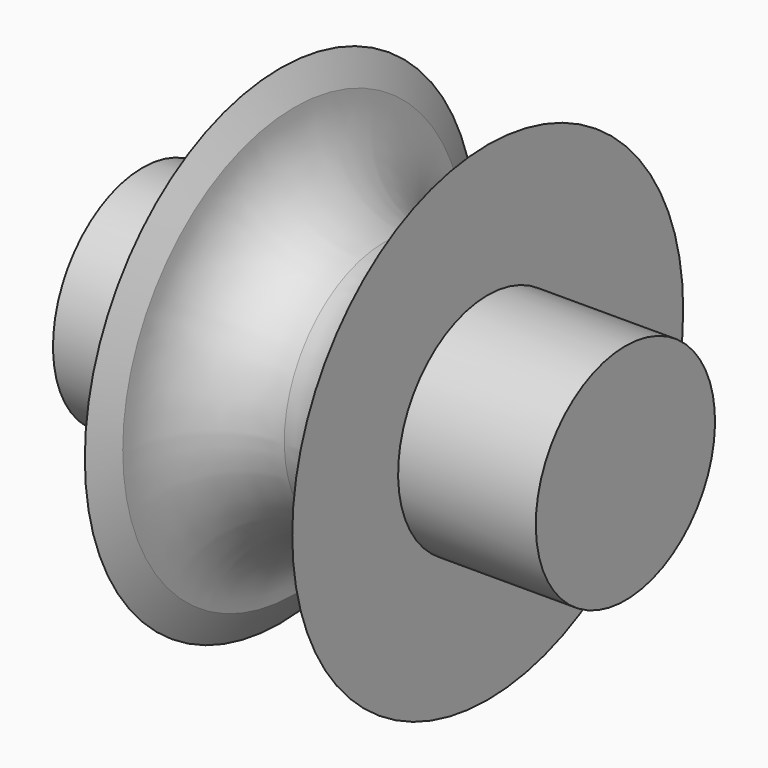
from build123d import *

# Parameters (mm, degrees)
F0_W = 14.6103731854
F0_H = 11.8872


# Not quite as in the source:
# - ends of sketch curves that miss each other by under 0.0002 mm in the source are joined


with BuildPart() as f1:
    # F0 (on Front) → F1 (revolve)
    with BuildSketch(Plane.XZ):
        with Locations((-13.6665977984, 5.9436)):
            Rectangle(F0_W, F0_H)
        with BuildLine():
            Line((-6.3614112057, 11.8872), (-6.3614112057, 0))
            Line((-6.3614112057, 0), (15.6496424236, 0))
            Line((15.6496424236, 0), (15.6496424236, 11.8872))
            Line((15.6496424236, 11.8872), (15.6496424236, 25.9283669293))
            Line((15.6496424236, 25.9283669293), (14.1691156089, 22.7533669293))
            ThreePointArc((14.1691156089, 22.7533669293), (11.3793089407, 16.0181760794), (4.6441191189, 13.2283669293))
            ThreePointArc((4.6441191189, 13.2283669293), (-2.0910777228, 16.0181760794), (-4.8808843911, 22.7533669293))
            Line((-4.8808843911, 22.7533669293), (-6.3614112057, 25.9283669293))
            Line((-6.3614112057, 25.9283669293), (-6.3614112057, 11.8872))
        make_face()
        with Locations((22.9548290163, 5.9436)):
            Rectangle(F0_W, F0_H)
    revolve(axis=Axis((4.6441156089, 0, 0), (1, 0, 0)))


solid = f1.part
